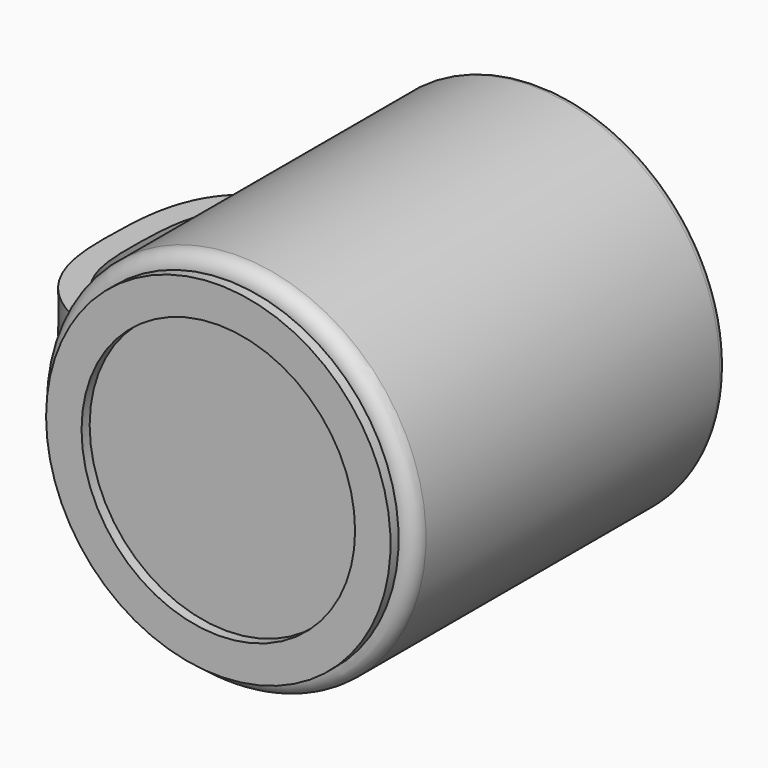
from build123d import *

# Parameters (mm, degrees)
F4_DEPTH = 8


# Not quite as in the source:
# - the dataset's text gives a spline's control points without its knots; the knots are read off the source's solid


with BuildPart() as f2:
    # F0 (on Top) → F2 (revolve)
    with BuildSketch(Plane.XY):
        with BuildLine():
            ThreePointArc((-45.635785236, 52.7449016869), (-46.6964454078, 52.3055618587), (-47.135785236, 51.2449016869))
            Line((-47.135785236, 51.2449016869), (-47.135785236, -21.2550983131))
            ThreePointArc((-47.135785236, -21.2550983131), (-46.2571055796, -23.3764186566), (-44.135785236, -24.2550983131))
            Line((-44.135785236, -24.2550983131), (-44.135785236, -26.2550983131))
            Line((-44.135785236, -26.2550983131), (-37.135785236, -26.2550983131))
            Line((-37.135785236, -26.2550983131), (-37.135785236, -24.2550983131))
            Line((-37.135785236, -24.2550983131), (-10.135785236, -24.2550983131))
            Line((-10.135785236, -24.2550983131), (-10.135785236, -17.2550983131))
            Line((-10.135785236, -17.2550983131), (-37.135785236, -17.2550983131))
            ThreePointArc((-37.135785236, -17.2550983131), (-39.2571055796, -16.3764186566), (-40.135785236, -14.2550983131))
            Line((-40.135785236, -14.2550983131), (-40.135785236, 51.2449016869))
            ThreePointArc((-40.135785236, 51.2449016869), (-40.5751250642, 52.3055618587), (-41.635785236, 52.7449016869))
            Line((-41.635785236, 52.7449016869), (-45.635785236, 52.7449016869))
        make_face()
    revolve(axis=Axis((-10.1351393387, 6.3089774922, 0), (0, 1, 0)))

    # F3 (on Top) → F4 (join)
    with BuildSketch(Plane.XY):
        with BuildLine():
            add(Edge.make_bspline(
                [(-47.2617670894, 37.8949455917), (-58.8366426528, 35.2238230407), (-60.0635604163, 15.0998280087), (-59.5044270158, -1.8380486872), (-47.0391735435, -6.2899244949)],
                knots=[0, 0, 0, 0, 0.49802797, 1, 1, 1, 1], degree=3))
            Line((-47.2617670894, 37.8949455917), (-47.1504703164, 42.766901808))
            Line((-47.1504703164, 42.766901808), (-48.3860635922, 42.766901808))
            add(Edge.make_bspline(
                [(-48.3860635922, 42.766901808), (-50.1690239959, 42.3554498044), (-52.6384721881, 41.4978707661), (-55.4934134363, 39.8722567285), (-57.3934460935, 38.4298265084), (-59.0339150802, 36.7973964039), (-60.8661224315, 34.4275406713), (-62.5095201326, 31.2277740356), (-63.6691903308, 27.2897617301), (-64.1762582918, 24.0296074922), (-64.408920176, 21.468947788), (-64.5181379905, 19.5803302862), (-64.5713544491, 18.0416416879), (-64.6002996245, 16.8352306226), (-64.6173421146, 15.9489680743), (-64.6317630804, 15.0622128366), (-64.6442959932, 13.8676880033), (-64.6415589323, 12.3578782321), (-64.5884434888, 10.5192391808), (-64.4207146322, 8.0343061588), (-63.9677821243, 4.8679436182), (-62.7988573666, 1.0147691249), (-60.7577790299, -2.7373998696), (-57.7249585965, -6.112176757), (-53.7532907219, -8.9028450806), (-50.5065385786, -10.3608901684), (-48.7208553836, -10.9986341046)],
                knots=[0, 0, 0, 0, 0.0625, 0.09375, 0.125, 0.15625, 0.1875, 0.25, 0.3125, 0.375, 0.40625, 0.4375, 0.46875, 0.484375, 0.5, 0.515625, 0.53125, 0.5625, 0.59375, 0.625, 0.6875, 0.75, 0.8125, 0.875, 0.9375, 1, 1, 1, 1], degree=3))
            Line((-48.7208553836, -10.9986341046), (-47.0391735435, -11.393670924))
            Line((-47.0391735435, -11.393670924), (-47.0391735435, -6.2899244949))
        make_face()
    extrude(amount=F4_DEPTH)


solid = f2.part
